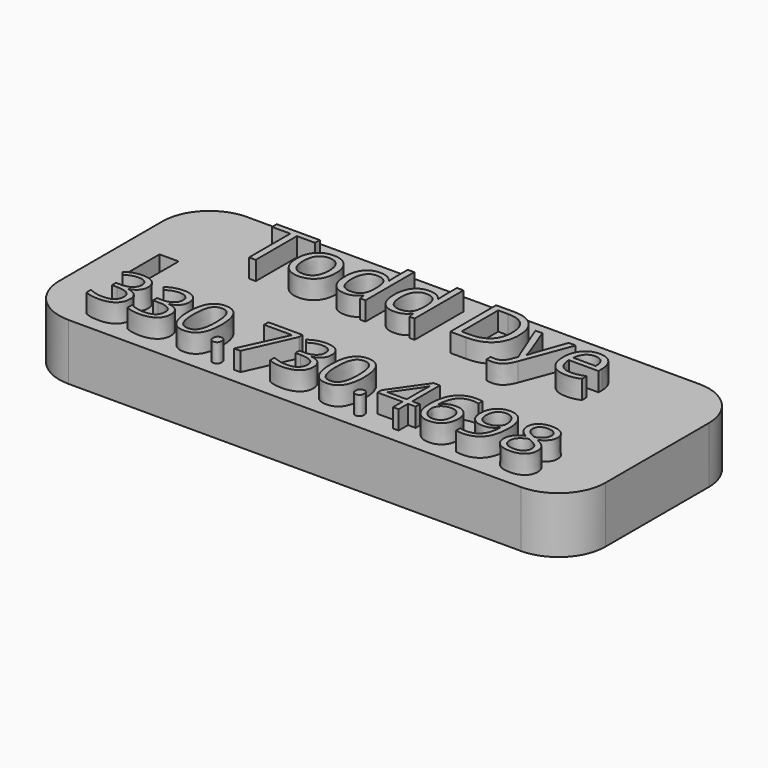
from build123d import *

# Parameters (mm, degrees)
F0_W         = 58.2218244672
F0_H         = 23.7748990767
F1_DEPTH     = 6
F2_R         = 5
F5_TEXT_SIZE = 7.6646706587
F4_TEXT_SIZE = 8.5560171606
F6_DEPTH     = 2
F7_W         = 2.0408891141
F7_H         = 4.1555203497
F8_DEPTH     = 6


# Not quite as in the source:
# - Text() gives the source's letters only with a copy of the font that has no kerning and outlines rounded to 1/6400 em; it was checked with that copy


with BuildPart() as f1:
    # F0 (on Top) → F1 (new body)
    with BuildSketch(Plane.XY):
        Rectangle(F0_W, F0_H)
    extrude(amount=F1_DEPTH)

    # F2
    f2_edges = [f1.edges().sort_by_distance(p)[0] for p in [
        (-29.110912, 11.88745, 3),
        (29.110912, 11.88745, 3),
        (29.110912, -11.88745, 3),
        (-29.110912, -11.88745, 3),
    ]]
    fillet(f2_edges, radius=F2_R)

    # F5 (on face) + F4 (on face) → F6 (join)
    with BuildSketch(Plane.XY.offset(6)):
        with Locations((-24, -10.2928760317)):
            Text('330.730.4698', F5_TEXT_SIZE, font='Open Sans', text_align=(TextAlign.LEFT, TextAlign.BOTTOM))
    with BuildSketch(Plane.XY.offset(6)):
        with Locations((-19.034464427, 3.3106910996)):
            Text('Todd Dye', F4_TEXT_SIZE, font='Open Sans', text_align=(TextAlign.LEFT, TextAlign.BOTTOM))
    extrude(amount=F6_DEPTH)

    # F7 (on face) → F8 (cut, through all)
    with BuildSketch(Plane.XY.offset(6)):
        with Locations((-24.5690140873, 0)):
            Rectangle(F7_W, F7_H)
    extrude(amount=-F8_DEPTH, mode=Mode.SUBTRACT)


solid = f1.part
